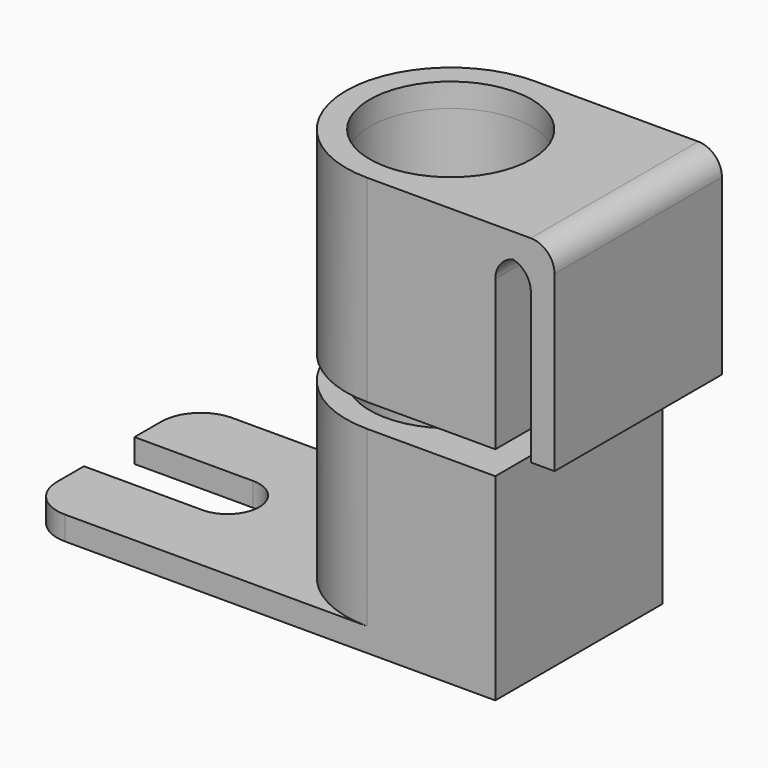
from build123d import *

# Parameters (mm, degrees)
F0_R        = 10.25
F0_W        = 4.5
F0_H        = 26.5
F0_W_2      = 3
F1_DEPTH    = 3
F2_DEPTH    = 22
F3_T1_DEPTH = 26.5
F3_T3_DEPTH = 41.5
F5_R        = 10.25
F6_DEPTH    = 22
F7_DEPTH    = 3
F8_R        = 5


# Not quite as in the source:
# - a fillet or chamfer that OpenCascade refuses, or shapes differently, is made with other operations: its cross-section is extruded or revolved along the edge and cut away or added


with BuildPart() as f1:
    # F0 (on Top) → F1 (new body)
    with BuildSketch(Plane.XY):
        with BuildLine():
            ThreePointArc((0, -13.25), (9.3691648507, -9.3691648507), (13.25, 0))
            ThreePointArc((13.25, 0), (9.3691648507, 9.3691648507), (0, 13.25))
            ThreePointArc((0, 13.25), (-13.25, 0), (0, -13.25))
        make_face()
        Circle(F0_R, mode=Mode.SUBTRACT)
        with BuildLine():
            Line((13.25, -13.25), (13.25, 0))
            ThreePointArc((13.25, 0), (9.3691648507, -9.3691648507), (0, -13.25))
            Line((0, -13.25), (13.25, -13.25))
        make_face()
        with BuildLine():
            ThreePointArc((0, 13.25), (9.3691648507, 9.3691648507), (13.25, 0))
            Line((13.25, 0), (13.25, 13.25))
            Line((13.25, 13.25), (0, 13.25))
        make_face()
        Polygon((13.25, 13.25), (13.25, 0), (13.25, -13.25), (16.25, -13.25), (16.25, 13.25), align=None)
        with Locations((18.5, 0)):
            Rectangle(F0_W, F0_H)
        with Locations((22.25, 0)):
            Rectangle(F0_W_2, F0_H)
    extrude(amount=F1_DEPTH)

    # F0 (on Top) → F2 (join)
    with BuildSketch(Plane.XY):
        with BuildLine():
            ThreePointArc((0, -13.25), (9.3691648507, -9.3691648507), (13.25, 0))
            ThreePointArc((13.25, 0), (9.3691648507, 9.3691648507), (0, 13.25))
            ThreePointArc((0, 13.25), (-13.25, 0), (0, -13.25))
        make_face()
        Circle(F0_R, mode=Mode.SUBTRACT)
        with BuildLine():
            ThreePointArc((0, 13.25), (9.3691648507, 9.3691648507), (13.25, 0))
            Line((13.25, 0), (13.25, 13.25))
            Line((13.25, 13.25), (0, 13.25))
        make_face()
        Polygon((13.25, 13.25), (13.25, 0), (13.25, -13.25), (16.25, -13.25), (16.25, 13.25), align=None)
        with Locations((22.25, 0)):
            Rectangle(F0_W_2, F0_H)
        with BuildLine():
            Line((13.25, -13.25), (13.25, 0))
            ThreePointArc((13.25, 0), (9.3691648507, -9.3691648507), (0, -13.25))
            Line((0, -13.25), (13.25, -13.25))
        make_face()
    extrude(amount=-F2_DEPTH)

    # F3: fillet of radius 3 on 3 edges, made by hand

    # F3_s2 → F3_t1 (join)
    with BuildSketch(Plane.XZ.offset(-13.25)):
        with BuildLine():
            ThreePointArc((16.25, -3), (17.1286796564, -0.8786796564), (19.25, 0))
            Line((19.25, 0), (16.25, 0))
            Line((16.25, 0), (16.25, -3))
        make_face()
        with BuildLine():
            ThreePointArc((17.75, 0), (19.8713203436, -0.8786796564), (20.75, -3))
            Line((20.75, -3), (20.75, 0))
            Line((20.75, 0), (17.75, 0))
        make_face()
    extrude(amount=F3_T1_DEPTH)

    # F3_s4 → F3_t3 (cut)
    with BuildSketch(Plane.XZ.offset(-20.75)):
        with BuildLine():
            ThreePointArc((20.75, 3), (22.8713203436, 2.1213203436), (23.75, 0))
            Line((23.75, 0), (23.75, 3))
            Line((23.75, 3), (20.75, 3))
        make_face()
    extrude(amount=F3_T3_DEPTH, mode=Mode.SUBTRACT)


with BuildPart() as f6:
    # F5 (on offset) → F6 (new body)
    with BuildSketch(Plane(origin=(0, 0, -47), x_dir=(1, 0, 0), z_dir=(0, 0, -1))):
        with BuildLine():
            Line((16.25, 13.25), (0, 13.25))
            ThreePointArc((0, 13.25), (-13.25, 0), (0, -13.25))
            Line((0, -13.25), (16.25, -13.25))
            Line((16.25, -13.25), (16.25, 13.25))
        make_face()
        Circle(F5_R, mode=Mode.SUBTRACT)
    extrude(amount=-F6_DEPTH)

    # F5 (on offset) → F7 (join)
    with BuildSketch(Plane(origin=(0, 0, -47), x_dir=(1, 0, 0), z_dir=(0, 0, -1))):
        with BuildLine():
            Line((16.25, 13.25), (0, 13.25))
            ThreePointArc((0, 13.25), (-13.25, 0), (0, -13.25))
            Line((0, -13.25), (16.25, -13.25))
            Line((16.25, -13.25), (16.25, 13.25))
        make_face()
        Circle(F5_R, mode=Mode.SUBTRACT)
        with BuildLine():
            ThreePointArc((0, -13.25), (-13.25, 0), (0, 13.25))
            Line((0, 13.25), (-43.25, 13.25))
            Line((-43.25, 13.25), (-43.25, 4))
            Line((-43.25, 4), (-28.25, 4))
            ThreePointArc((-28.25, 4), (-24.25, 0), (-28.25, -4))
            Line((-28.25, -4), (-43.25, -4))
            Line((-43.25, -4), (-43.25, -13.25))
            Line((-43.25, -13.25), (0, -13.25))
        make_face()
    extrude(amount=F7_DEPTH)

    # F8
    f8_edges = [f6.edges().sort_by_distance(p)[0] for p in [
        (-43.25, -13.25, -48.5),
        (-43.25, 13.25, -48.5),
    ]]
    fillet(f8_edges, radius=F8_R)


solid = Compound([f1.part, f6.part])
